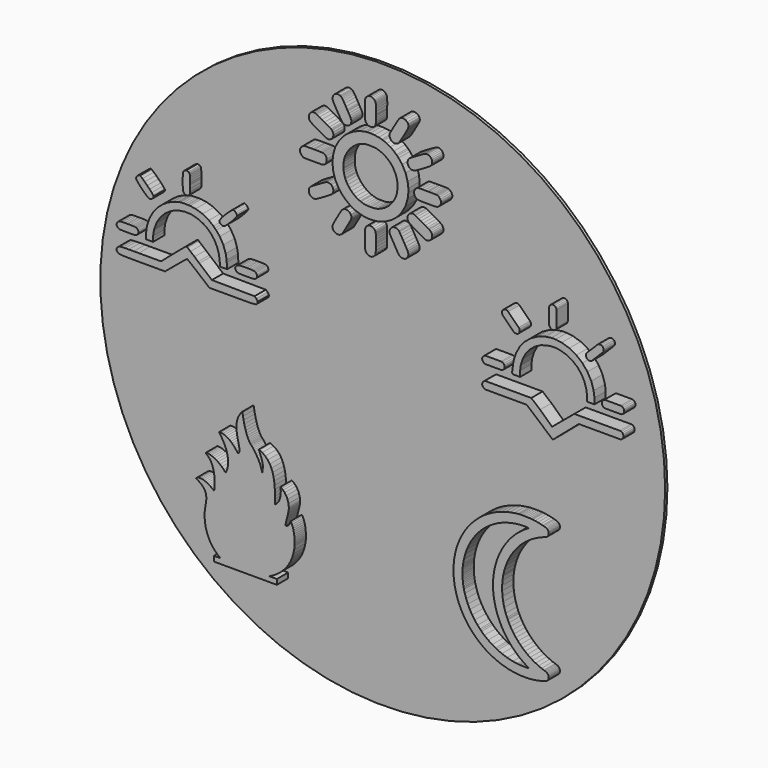
from build123d import *

# Parameters (mm, degrees)
F0_R      = 2.54
F1_DEPTH  = 0.0254
F7_DEPTH  = 0.127
F8_DEPTH  = 0.127
F9_DEPTH  = 0.127
F10_DEPTH = 0.127
F11_DEPTH = 0.127


# Not quite as in the source:
# - a feature names something its author has since deleted; it is built from what else it names


with BuildPart() as f1:
    # F0 (on Front) → F1 (new body)
    with BuildSketch(Plane.XZ):
        Circle(F0_R)
    extrude(amount=F1_DEPTH)


with BuildPart() as f7:
    # F2 (on face) → F7 (new body)
    with BuildSketch(Plane.XZ.offset(0.0254)):
        Polygon((1.2692778416, 0.5493445328), (1.270369884, 0.5471772229), (1.3371176617, 0.5471772229), (1.3371176617, 0.5513474493), (1.3371176617, 0.5638111588), (1.3371176617, 0.5764996513), (1.3371176617, 0.5807235571), (1.3371176617, 0.595958471), (1.3431767355, 0.6416296629), (1.3605789593, 0.6982145687), (1.3881735787, 0.74934765), (1.4247930644, 0.793831183), (1.4692464026, 0.8304707985), (1.520372774, 0.8581023226), (1.5770180693, 0.8755582259), (1.6227597155, 0.8816206547), (1.6380080493, 0.8816206547), (1.6532463181, 0.8816206547), (1.6989846094, 0.8755582259), (1.7556533894, 0.8581560021), (1.8067797608, 0.8305613827), (1.8512263891, 0.7939586718), (1.8878525848, 0.7495086886), (1.9154472041, 0.6983588324), (1.932846073, 0.6417168921), (1.9389252766, 0.5959786008), (1.9389252766, 0.5807235571), (1.9389252766, 0.5765768156), (1.9389252766, 0.5640862663), (1.9389252766, 0.5514179036), (1.9389252766, 0.5471772229), (2.0056723833, 0.5471772229), (2.0056723833, 0.5513474493), (2.0056723833, 0.5638111588), (2.0056723833, 0.5764996513), (2.0056723833, 0.5807235571), (2.0056723833, 0.599092012), (1.9981002185, 0.6541302771), (1.9764170543, 0.7228064909), (1.9422198561, 0.7852022029), (1.8970586195, 0.8397741274), (1.84249005, 0.8849487839), (1.7800775632, 0.9191325622), (1.7113979944, 0.9408123714), (1.6563597293, 0.9483677614), (1.6380080493, 0.9483677614), (1.6196630792, 0.9483677614), (1.5646181041, 0.9408123714), (1.4959452453, 0.9191325622), (1.4335327585, 0.8849487839), (1.378960834, 0.8397741274), (1.3338029524, 0.7852022029), (1.2996020637, 0.7228064909), (1.277923932, 0.6541302771), (1.270369884, 0.599092012), (1.270369884, 0.5807235571), (1.2692959584, 0.5785226975), (1.2666203707, 0.5716047516), (1.2653827227, 0.5638111588), (1.2666203707, 0.5561148601), align=None)
    extrude(amount=F7_DEPTH)


with BuildPart() as f7b:
    # F2 (on face) → F7, piece 2 (new body)
    with BuildSketch(Plane.XZ.offset(0.0254)):
        Polygon((1.1833466872, 0.9815651788), (1.2770137289, 0.8879179314), (1.2793071857, 0.8856063578), (1.2880441958, 0.8804564805), (1.3004213471, 0.8779570286), (1.3127803816, 0.8804564805), (1.3215173917, 0.8856063578), (1.3238474176, 0.8879179314), (1.3261589912, 0.89022615), (1.331309875, 0.898965844), (1.3337861775, 0.9113255495), (1.331309875, 0.9237020299), (1.3261589912, 0.9324215941), (1.3238474176, 0.9347331677), (1.2301803758, 1.028400545), (1.2278503499, 1.0307322484), (1.2191136753, 1.0358787707), (1.2067546408, 1.0383715126), (1.1943952708, 1.0358787707), (1.1856585962, 1.0307322484), (1.1833466872, 1.028400545), (1.1810351136, 1.0260856164), (1.175866113, 1.0173660522), (1.1733904814, 1.0049895718), (1.175866113, 0.9926332213), (1.1810169967, 0.9838968822), align=None)
    extrude(amount=F7_DEPTH)


with BuildPart() as f7c:
    # F2 (on face) → F7, piece 3 (new body)
    with BuildSketch(Plane.XZ.offset(0.0254)):
        Polygon((1.0261737742, 0.5471772229), (1.0295773901, 0.5471772229), (1.1630883783, 0.5471772229), (1.1664916588, 0.5471772229), (1.1767212945, 0.5495827356), (1.1873149444, 0.5563530629), (1.1941768623, 0.5669446998), (1.1966343771, 0.577284714), (1.1966343771, 0.5807235571), (1.1966343771, 0.5841791751), (1.1942318838, 0.5945191893), (1.1874420977, 0.6051141812), (1.1768669002, 0.6118878634), (1.166528228, 0.6142732463), (1.1630883783, 0.6142732463), (1.0295773901, 0.6142732463), (1.0261553218, 0.6142732463), (1.0159260216, 0.610958537), (1.0053327072, 0.6026214393), (0.9984704538, 0.5917177903), (0.9960313914, 0.5834712767), (0.9960313914, 0.5807235571), (0.9960860774, 0.577284714), (0.9986160595, 0.5669446998), (1.0054598606, 0.5563530629), (1.0159807076, 0.5495827356), align=None)
    extrude(amount=F7_DEPTH)


with BuildPart() as f7d:
    # F2 (on face) → F7, piece 4 (new body)
    with BuildSketch(Plane.XZ.offset(0.0254)):
        Polygon((2.2362157826, 0.4133206729), (2.232830619, 0.4133206729), (1.8249804672, 0.4133206729), (1.7445987668, 0.3465749082), (1.6243969404, 0.2462821383), (1.5174405312, 0.3465749082), (1.4374278774, 0.4133206729), (1.0295773901, 0.4133206729), (1.0268652333, 0.4133206729), (1.0187290981, 0.41093529), (1.0078261201, 0.4041649627), (0.9993987737, 0.3935733259), (0.9960313914, 0.3832333116), (0.9960313914, 0.3797743387), (0.9960313914, 0.3763348246), (0.9993440877, 0.3659964878), (1.0076805145, 0.3554025025), (1.0185834925, 0.3486315042), (1.0268289996, 0.3462290109), (1.0295773901, 0.3462290109), (1.3972387047, 0.3462290109), (1.631019649, 0.1456260253), (1.8648240781, 0.3462290109), (2.2324850572, 0.3462290109), (2.2358869957, 0.3462290109), (2.2461162959, 0.3486315042), (2.2567112877, 0.3554025025), (2.2635721992, 0.3659964878), (2.2660313914, 0.3763348246), (2.2660313914, 0.3797743387), (2.2660313914, 0.3832333116), (2.2636258787, 0.3935733259), (2.2568924561, 0.4041649627), (2.2464081782, 0.41093529), align=None)
    extrude(amount=F7_DEPTH)


with BuildPart() as f7e:
    # F2 (on face) → F7, piece 5 (new body)
    with BuildSketch(Plane.XZ.offset(0.0254)):
        Polygon((2.072416135, 0.5830888102), (2.072416135, 0.5803779953), (2.072416135, 0.5769760569), (2.0748015179, 0.5667232718), (2.081591975, 0.556131635), (2.0921634821, 0.5492707235), (2.1025034963, 0.5468148863), (2.1059624692, 0.5468148863), (2.2394768124, 0.5468148863), (2.2428787509, 0.5468148863), (2.2531046962, 0.549217044), (2.263703043, 0.5560075011), (2.2705605994, 0.5665790082), (2.2730197917, 0.5769391522), (2.2730197917, 0.5803779953), (2.2730197917, 0.5838336133), (2.2706176339, 0.5941736275), (2.2638271768, 0.6047518445), (2.2532556698, 0.6115423016), (2.2429156555, 0.6139209746), (2.2394768124, 0.6139209746), (2.1059624692, 0.6139209746), (2.1025034963, 0.6139209746), (2.0921634821, 0.6105592957), (2.081591975, 0.6021282589), (2.0748015179, 0.5912246099), align=None)
    extrude(amount=F7_DEPTH)


with BuildPart() as f7f:
    # F2 (on face) → F7, piece 6 (new body)
    with BuildSketch(Plane.XZ.offset(0.0254)):
        Polygon((1.984227422, 0.8856063578), (1.9853915962, 0.8879179314), (2.0790623284, 0.9815651788), (2.081373902, 0.9838968822), (2.0865204244, 0.9926332213), (2.0890198762, 1.0049895718), (2.0865204244, 1.0173492773), (2.081373902, 1.0260856164), (2.0790623284, 1.028400545), (2.076730625, 1.0307322484), (2.067994286, 1.0358787707), (2.0556345805, 1.0383715126), (2.043274875, 1.0358787707), (2.0345385359, 1.0307322484), (2.0322269623, 1.028400545), (1.9385763599, 0.9347331677), (1.9362647863, 0.9324215941), (1.9310981342, 0.9237020299), (1.9286053922, 0.9113255495), (1.9310981342, 0.898965844), (1.9362480114, 0.89022615), (1.9385763599, 0.8879179314), (1.9410556819, 0.8854989988), (1.9507012176, 0.8804564805), (1.9645874339, 0.8779570286), (1.9771886972, 0.8804564805), align=None)
    extrude(amount=F7_DEPTH)


with BuildPart() as f7g:
    # F2 (on face) → F7, piece 7 (new body)
    with BuildSketch(Plane.XZ.offset(0.0254)):
        Polygon((1.6286208462, 1.0147659513), (1.6313886956, 1.0147659513), (1.6347906341, 1.0147659513), (1.6450165793, 1.017164754), (1.6556149262, 1.0239552111), (1.6624724826, 1.0345334281), (1.6649316749, 1.0448902172), (1.6649316749, 1.0483290603), (1.6649316749, 1.1818199187), (1.6649316749, 1.185245342), (1.6625295171, 1.1954746422), (1.65573906, 1.2060662791), (1.6451675529, 1.2129305455), (1.6348275387, 1.2153696079), (1.6313886956, 1.2153696079), (1.6286577509, 1.2153696079), (1.6205219513, 1.212984225), (1.6096183023, 1.2062138977), (1.6011872654, 1.1956189059), (1.5978188766, 1.1852788917), (1.5978188766, 1.1818199187), (1.5978188766, 1.0483290603), (1.5978188766, 1.0449237669), (1.6011335859, 1.0346776918), (1.6094874585, 1.0240860549), (1.6203709777, 1.0172217885), align=None)
    extrude(amount=F7_DEPTH)


with BuildPart() as f8:
    # F3 (on face) → F8 (new body)
    with BuildSketch(Plane.XZ.offset(0.0254)):
        Polygon((-1.7690962786, 0.5183341948), (-1.7800488386, 0.5088888379), (-1.8924155646, 0.4123955589), (-2.0774647861, 0.4123955589), (-2.0923647631, 0.4123955589), (-2.1369972622, 0.412351013), (-2.1824724545, 0.4121291011), (-2.2159962788, 0.4116194801), (-2.2396766941, 0.4106881038), (-2.2556404589, 0.4092471066), (-2.2660171921, 0.4071403735), (-2.2728903321, 0.404258379), (-2.2770809123, 0.4014867275), (-2.2783890894, 0.4004666682), (-2.281249424, 0.3982716607), (-2.288521842, 0.389890909), (-2.2924463731, 0.3786935512), (-2.2902292971, 0.367208893), (-2.2843091932, 0.3581399282), (-2.2818035908, 0.3556347344), (-2.2808280773, 0.3546588123), (-2.2775243276, 0.3520649355), (-2.2712274229, 0.3493153525), (-2.2606071179, 0.3473201885), (-2.2434234505, 0.3459233284), (-2.2173931388, 0.3450360893), (-2.1802108326, 0.3445485369), (-2.1295916152, 0.3443486936), (-2.0798596369, 0.3442824878), (-2.0632746822, 0.3442824878), (-1.8560996549, 0.3442824878), (-1.7590264623, 0.4254548519), (-1.7495614889, 0.4333259827), (-1.721068486, 0.4568282146), (-1.6894531861, 0.4827252974), (-1.6674990249, 0.5004189945), (-1.6590067042, 0.5070485627), (-1.6585653324, 0.5071813829), (-1.6580136176, 0.5074699093), (-1.6492311358, 0.5013724393), (-1.6268560367, 0.4841221574), (-1.594799365, 0.4582696206), (-1.5659753332, 0.434545068), (-1.5563959301, 0.4265856629), (-1.4576430725, 0.3442824878), (-1.2493360083, 0.3442824878), (-1.233078813, 0.3442824878), (-1.1842581858, 0.344326625), (-1.1341052695, 0.3445264683), (-1.0968093509, 0.3449919521), (-1.0703147815, 0.3457900995), (-1.0525986071, 0.3470320707), (-1.0415561381, 0.3488498687), (-1.0351725939, 0.351311334), (-1.0321810738, 0.3535946158), (-1.0313596318, 0.3545039235), (-1.0292304214, 0.3568317511), (-1.0240402158, 0.364968931), (-1.0224463731, 0.3747914974), (-1.0265903641, 0.3848351583), (-1.0337749164, 0.3934386393), (-1.036484449, 0.3959438331), (-1.0512254504, 0.4095572929), (-1.4349369446, 0.412972203), (-1.5473314607, 0.5088888379), (-1.5582186322, 0.5183562634), (-1.5910517913, 0.5464928995), (-1.6276366109, 0.5771551631), (-1.6531789615, 0.5978219899), (-1.6610746129, 0.6053825256), (-1.6636901496, 0.6053825256), (-1.6663015995, 0.6053825256), (-1.6741277758, 0.5978219899), (-1.6995189156, 0.5771551631), (-1.7360792146, 0.5464928995), align=None)
    extrude(amount=F8_DEPTH)


with BuildPart() as f8b:
    # F3 (on face) → F8, piece 2 (new body)
    with BuildSketch(Plane.XZ.offset(0.0254)):
        Polygon((-1.2100866107, 0.600081977), (-1.2112840361, 0.5991297582), (-1.2141447793, 0.5969351594), (-1.2214233275, 0.5885531817), (-1.2253425458, 0.5773554152), (-1.2231234264, 0.5658715744), (-1.2172057746, 0.5568030182), (-1.2147005809, 0.5542978245), (-1.2137933166, 0.5533864734), (-1.2108426642, 0.5508812796), (-1.2063839915, 0.5482224231), (-1.2006420711, 0.5462264417), (-1.1928608494, 0.544807513), (-1.1823087936, 0.5438544768), (-1.168246197, 0.5432999013), (-1.1499823947, 0.5430338522), (-1.1325522946, 0.5429451691), (-1.1267204651, 0.5429451691), (-1.1209172431, 0.5429451691), (-1.1034830563, 0.5430338522), (-1.0852110803, 0.5432999013), (-1.0711566574, 0.5438544768), (-1.0606086883, 0.544807513), (-1.052819293, 0.5462264417), (-1.0470814594, 0.5482224231), (-1.0426268735, 0.5508812796), (-1.0396517005, 0.5533864734), (-1.0387444362, 0.5542978245), (-1.0371914612, 0.5558712333), (-1.0307384418, 0.5656508884), (-1.0273913722, 0.574163643), (-1.0273913722, 0.5769998657), (-1.0273913722, 0.579840175), (-1.0307384418, 0.5883529296), (-1.0371914612, 0.5981530187), (-1.0387444362, 0.5997059936), (-1.0396721343, 0.6006377786), (-1.0426268735, 0.6031429723), (-1.0470119842, 0.6058034636), (-1.0526435617, 0.6077978103), (-1.0601795768, 0.6092159216), (-1.0703352154, 0.6101722272), (-1.0837766219, 0.610723942), (-1.1012026352, 0.6109936692), (-1.1177867726, 0.6110590576), (-1.1233039203, 0.6110590576), (-1.1288047209, 0.6110590576), (-1.1452826021, 0.6109936692), (-1.1626840948, 0.610723942), (-1.1762562782, 0.6101477066), (-1.1866734704, 0.6091505332), (-1.1946835516, 0.6076670335), (-1.2009771868, 0.605558257), (-1.2062777353, 0.6027424683), align=None)
    extrude(amount=F8_DEPTH)


with BuildPart() as f8c:
    # F3 (on face) → F8, piece 3 (new body)
    with BuildSketch(Plane.XZ.offset(0.0254)):
        Polygon((-1.3050305929, 0.9794451415), (-1.3106172158, 0.9737481756), (-1.319975933, 0.9644180658), (-1.3470671718, 0.9354183026), (-1.3649876849, 0.9101211586), (-1.3665120524, 0.8932223394), (-1.3574884508, 0.8825803745), (-1.3537653978, 0.8800915279), (-1.3517914849, 0.8788328008), (-1.3401523466, 0.8745089917), (-1.3285132083, 0.8738673679), (-1.3265147748, 0.8744149959), (-1.3237194199, 0.8751097478), (-1.3160934958, 0.8803367344), (-1.3002613252, 0.8932427733), (-1.2811270395, 0.9109834684), (-1.2607503739, 0.9313356133), (-1.2412646255, 0.9521781714), (-1.2247663104, 0.9713369777), (-1.2133274241, 0.9866337806), (-1.2090240489, 0.9935976471), (-1.2090240489, 0.9959025888), (-1.2090240489, 0.9987837659), (-1.212526416, 1.0073864296), (-1.2212394226, 1.0188294027), (-1.2325066643, 1.0276077977), (-1.2408845553, 1.031089731), (-1.2436594763, 1.031089731), (-1.2457886866, 1.031089731), (-1.2521272763, 1.0266106244), (-1.2675548561, 1.0143502961), (-1.2878048316, 0.9961477954), align=None)
    extrude(amount=F8_DEPTH)


with BuildPart() as f8d:
    # F3 (on face) → F8, piece 4 (new body)
    with BuildSketch(Plane.XZ.offset(0.0254)):
        Polygon((-1.6824198445, 1.1991093565), (-1.6858159554, 1.1956928117), (-1.6867232197, 1.1947855474), (-1.6892488473, 1.1918348951), (-1.6919134253, 1.1873803091), (-1.6939077721, 1.1816343019), (-1.6953299701, 1.1738530802), (-1.696282189, 1.1633010244), (-1.6968339037, 1.1492425146), (-1.6970995442, 1.1309746255), (-1.6971690194, 1.1135445254), (-1.6971690194, 1.1077167827), (-1.6971690194, 1.1019094739), (-1.6970995442, 1.0844752871), (-1.6968339037, 1.0662114847), (-1.696282189, 1.052152975), (-1.6953299701, 1.0416009191), (-1.6939077721, 1.0338115238), (-1.6919134253, 1.0280736902), (-1.6892488473, 1.0236191043), (-1.6867477403, 1.0206684519), (-1.6858159554, 1.019736667), (-1.6831309435, 1.0170516551), (-1.6730897346, 1.0109991397), (-1.6597178033, 1.0085348137), (-1.6471877478, 1.0122415196), (-1.6388956791, 1.0191399977), (-1.6369912414, 1.0219966542), (-1.6355526962, 1.0243669843), (-1.6326020439, 1.0323770654), (-1.6302071931, 1.0483359261), (-1.629496094, 1.0739927064), (-1.6299415526, 1.1035482711), (-1.6301826724, 1.1133892279), (-1.6303420567, 1.1192210574), (-1.6308242963, 1.1366756781), (-1.6315190482, 1.1549640011), (-1.6323568373, 1.1689979902), (-1.6334643536, 1.1794683106), (-1.6349519401, 1.1870043257), (-1.6369054191, 1.1923457421), (-1.6394514806, 1.1961587042), (-1.6418258975, 1.1984636459), (-1.6426677734, 1.1991093565), (-1.6465011694, 1.2018148023), (-1.6649039221, 1.2065595493), align=None)
    extrude(amount=F8_DEPTH)


with BuildPart() as f8e:
    # F3 (on face) → F8, piece 5 (new body)
    with BuildSketch(Plane.XZ.offset(0.0254)):
        Polygon((-2.1042932451, 1.021305989), (-2.1058454027, 1.019736667), (-2.1074192202, 1.0181877788), (-2.113871831, 1.0080321402), (-2.1171972407, 0.9989390634), (-2.1171972407, 0.9959025888), (-2.1171972407, 0.9933524405), (-2.1125857225, 0.9857019957), (-2.1002575537, 0.9693834987), (-2.0825421967, 0.9492724736), (-2.0617229333, 0.927653428), (-2.0401051138, 0.9068313038), (-2.0199944973, 0.8891192163), (-2.0036760004, 0.8767894128), (-1.9960263729, 0.8721590955), (-1.9934545647, 0.8721590955), (-1.9905276156, 0.8721590955), (-1.9817475859, 0.8753059131), (-1.9703512021, 0.883172957), (-1.9617039925, 0.8934879799), (-1.9582674225, 0.9013386768), (-1.9582674225, 0.9039542135), (-1.9582674225, 0.9062591552), (-1.963167467, 0.9131780671), (-1.9761376683, 0.9293167459), (-1.9946961273, 0.9499140974), (-2.0163805612, 0.9724199734), (-2.0386857764, 0.9943087461), (-2.059084102, 1.0130588748), (-2.0751144812, 1.0261651658), (-2.0819880299, 1.031089731), (-2.0842717204, 1.031089731), (-2.0869326203, 1.031089731), (-2.0948478882, 1.0277630952), align=None)
    extrude(amount=F8_DEPTH)


with BuildPart() as f8f:
    # F3 (on face) → F8, piece 6 (new body)
    with BuildSketch(Plane.XZ.offset(0.0254)):
        Polygon((-2.2796972664, 0.5990848037), (-2.2806727799, 0.5979977212), (-2.2831563137, 0.5953617506), (-2.2894086724, 0.5863136284), (-2.2925350561, 0.5755163659), (-2.2900294537, 0.5650501324), (-2.2841759643, 0.5566681546), (-2.2818035908, 0.5542978245), (-2.2808946918, 0.5533864734), (-2.2779456742, 0.5508812796), (-2.2734890448, 0.5482224231), (-2.2677467157, 0.5462264417), (-2.259964268, 0.544807513), (-2.2494101688, 0.5438544768), (-2.235352885, 0.5432999013), (-2.2170833612, 0.5430338522), (-2.1996553045, 0.5429451691), (-2.1938242924, 0.5429451691), (-2.1880157576, 0.5429451691), (-2.1705877009, 0.5430338522), (-2.1523181771, 0.5432999013), (-2.1382608933, 0.5438544768), (-2.1277072027, 0.544807513), (-2.119924755, 0.5462264417), (-2.1141816086, 0.5482224231), (-2.1097253879, 0.5508812796), (-2.1067547104, 0.5533864734), (-2.1058454027, 0.5542978245), (-2.1034726205, 0.5566926752), (-2.0978631116, 0.565385248), (-2.0952026204, 0.5769998657), (-2.0978631116, 0.5886185701), (-2.1034726205, 0.5973315767), (-2.1058454027, 0.5997059936), (-2.106776779, 0.6006377786), (-2.1097253879, 0.6031429723), (-2.11415954, 0.6058034636), (-2.1198577319, 0.6077978103), (-2.1275739738, 0.6092159216), (-2.1379952529, 0.6101722272), (-2.1518306247, 0.610723942), (-2.1698340994, 0.6109936692), (-2.1869956982, 0.6110590576), (-2.1926938901, 0.6110590576), (-2.198702677, 0.6110590576), (-2.2167057431, 0.6110141031), (-2.235264202, 0.6107934172), (-2.2492328027, 0.6102376156), (-2.259476307, 0.6092159216), (-2.2668594767, 0.6076220789), (-2.2722916194, 0.6053171372), (-2.27659336, 0.602145799), align=None)
    extrude(amount=F8_DEPTH)


with BuildPart() as f8g:
    # F3 (on face) → F8, piece 7 (new body)
    with BuildSketch(Plane.XZ.offset(0.0254)):
        Polygon((-1.7252819521, 0.9353038729), (-1.728387902, 0.9345927738), (-1.7422665936, 0.9316257744), (-1.7830607925, 0.919075285), (-1.8327723369, 0.8967247066), (-1.8785360556, 0.8669239353), (-1.911351233, 0.8391665521), (-1.9213728253, 0.8290068267), (-1.9336343796, 0.8166851968), (-1.9655623178, 0.774865217), (-1.9985765212, 0.7138046954), (-2.0192408958, 0.6484857531), (-2.026380085, 0.5982878823), (-2.026380085, 0.5815484474), (-2.026380085, 0.5429451691), (-1.9639431371, 0.5429451691), (-1.9639431371, 0.5701953835), (-1.963899, 0.5874456654), (-1.9560724151, 0.6391270358), (-1.9340773861, 0.7022064248), (-1.8998653487, 0.7578805756), (-1.8552536922, 0.8045556453), (-1.8021296898, 0.8406745724), (-1.7423769365, 0.8646639481), (-1.6778140478, 0.8749258429), (-1.6268110821, 0.8730867936), (-1.6103168538, 0.8698991083), (-1.5976151537, 0.8674143484), (-1.5601884583, 0.8560367638), (-1.514800723, 0.8351942057), (-1.4745337181, 0.8078577604), (-1.4398369891, 0.7744687997), (-1.4111437341, 0.7355340839), (-1.388842197, 0.6914990715), (-1.3733655759, 0.6428541756), (-1.3662014574, 0.6033432244), (-1.3651184618, 0.5900612021), (-1.3611502022, 0.5429451691), (-1.2981321148, 0.5429451691), (-1.3015486596, 0.595737734), (-1.3024804446, 0.6126324664), (-1.3110422405, 0.6629856347), (-1.3319215796, 0.7245120488), (-1.364292933, 0.780852344), (-1.396288303, 0.8205390266), (-1.4082666438, 0.8324233715), (-1.4206822695, 0.8446387452), (-1.461832018, 0.8773452143), (-1.5188139371, 0.9094100596), (-1.5806754668, 0.9292554443), (-1.6318255564, 0.9368364139), (-1.6489205408, 0.9374330832), (-1.6548872339, 0.9376537691), (-1.672754619, 0.937874455), (-1.6956814329, 0.9375229923), (-1.7151058797, 0.9364113892), align=None)
    extrude(amount=F8_DEPTH)


with BuildPart() as f9:
    # F4 (on face) → F9 (new body)
    with BuildSketch(Plane.XZ.offset(0.0254)):
        Polygon((-0.4048340655, 1.5237536493), (-0.4071004206, 1.522699946), (-0.4093578459, 1.5216623162), (-0.4159175954, 1.5180654375), (-0.4318374447, 1.5091911127), (-0.452495387, 1.4974378561), (-0.4754977298, 1.4841915556), (-0.4984904286, 1.4708291692), (-0.5190706826, 1.4587312267), (-0.5348837329, 1.4492621846), (-0.5414336597, 1.4452813292), (-0.5435266002, 1.4438168603), (-0.5464139258, 1.4417648178), (-0.5539329024, 1.4339727712), (-0.5606573153, 1.4224231116), (-0.5638062808, 1.4098858284), (-0.5634960634, 1.397094942), (-0.5598434635, 1.384780901), (-0.5529443858, 1.3736759399), (-0.5429258107, 1.3644997916), (-0.5333044281, 1.3591526939), (-0.529884, 1.3579882625), (-0.5278783919, 1.3573113921), (-0.521434907, 1.3564005638), (-0.5117456588, 1.3567881123), (-0.5014554425, 1.3590848283), (-0.4936555378, 1.3619726897), (-0.4911846929, 1.3632032008), (-0.487871064, 1.3648498354), (-0.4780750167, 1.3701308534), (-0.4599659648, 1.380246405), (-0.4388240333, 1.3923943538), (-0.4166248267, 1.4054084824), (-0.395347164, 1.4181029281), (-0.3769573627, 1.4293025439), (-0.36343067, 1.4378571859), (-0.3582371629, 1.4412004614), (-0.3567459049, 1.4425774194), (-0.3528597043, 1.4462118028), (-0.3446443905, 1.4608118442), (-0.341960126, 1.4816448084), (-0.3483448536, 1.5017383943), (-0.3589836849, 1.5147810979), (-0.3634413856, 1.5177386109), (-0.3657648907, 1.5192691596), (-0.3736158731, 1.5224963491), (-0.3854637844, 1.525053812), (-0.3972170409, 1.5252074027), align=None)
    extrude(amount=F9_DEPTH)


with BuildPart() as f9b:
    # F4 (on face) → F9, piece 2 (new body)
    with BuildSketch(Plane.XZ.offset(0.0254)):
        Polygon((-0.6034937473, 1.7449509729), (-0.6047923027, 1.7447009417), (-0.6085225909, 1.7439347743), (-0.6190451577, 1.7383840797), (-0.6315251123, 1.7268719248), (-0.6403713979, 1.7124344038), (-0.6437336044, 1.7010972708), (-0.6437336044, 1.6973200124), (-0.6436852055, 1.6937552806), (-0.640652326, 1.683066443), (-0.6328524213, 1.6690164705), (-0.6219326619, 1.6575257468), (-0.6128150924, 1.6518178896), (-0.6095011062, 1.6509374223), (-0.6085709899, 1.6506266691), (-0.6003253151, 1.6501033894), (-0.5803265625, 1.649483669), (-0.5524696836, 1.6490961205), (-0.5279073241, 1.6489496736), (-0.5197102269, 1.6489496736), (-0.5129565246, 1.6489496736), (-0.4926866666, 1.6489693189), (-0.4721064126, 1.6490461142), (-0.4569423721, 1.6492604267), (-0.4461678095, 1.6496676206), (-0.4387365224, 1.6503462769), (-0.4336305263, 1.6513642614), (-0.429792546, 1.6527769382), (-0.4270797065, 1.6541646119), (-0.4261992392, 1.6546575307), (-0.4216450978, 1.6570506873), (-0.4102686742, 1.6686467813), (-0.4019854948, 1.6878706156), (-0.4020337151, 1.708898247), (-0.4078469426, 1.7242376666), (-0.4110634165, 1.7283256782), (-0.4116831369, 1.7291097048), (-0.4138155466, 1.7312313989), (-0.4176142363, 1.7344693041), (-0.4219254901, 1.7376071968), (-0.4251026734, 1.7396431659), (-0.4261992392, 1.7402343113), (-0.4270904221, 1.7406879395), (-0.4298229069, 1.7419684569), (-0.4337073216, 1.7432954086), (-0.438804388, 1.7442741025), (-0.4460713688, 1.7449813339), (-0.4564673126, 1.7454546074), (-0.4709532326, 1.7457850059), (-0.490477283, 1.7459993184), (-0.5096139635, 1.7461439794), (-0.5159894041, 1.7461814841), (-0.5238862852, 1.7462314903), (-0.5475574617, 1.7462011294), (-0.574813194, 1.7459118075), (-0.5948607027, 1.7453885277), align=None)
    extrude(amount=F9_DEPTH)


with BuildPart() as f9c:
    # F4 (on face) → F9, piece 3 (new body)
    with BuildSketch(Plane.XZ.offset(0.0254)):
        Polygon((-0.5287988643, 2.0373857827), (-0.530872338, 2.0366499763), (-0.5360076235, 2.0348568948), (-0.5497664882, 2.0248181385), (-0.5611029068, 2.0068837514), (-0.5638353916, 1.9857900403), (-0.5596980882, 1.9691736752), (-0.5569172044, 1.9644641572), (-0.5563648139, 1.9635140383), (-0.5544463595, 1.9607922692), (-0.5509777112, 1.9570525155), (-0.5457358052, 1.9527412617), (-0.5379746554, 1.9473530874), (-0.5269288088, 1.9403861441), (-0.5118229899, 1.9313260818), (-0.4918921029, 1.9196799815), (-0.472765245, 1.908616097), (-0.4663799817, 1.9049317073), (-0.4617001103, 1.9022581585), (-0.4476126331, 1.8942553713), (-0.4325732511, 1.8858453903), (-0.4207146243, 1.8794499471), (-0.4114706103, 1.8747993651), (-0.4042911404, 1.8716400412), (-0.3986136442, 1.8697112284), (-0.3938666216, 1.8687414642), (-0.3905787102, 1.8684717876), (-0.3894857162, 1.8684717876), (-0.3872390065, 1.8684717876), (-0.3804631586, 1.8697987393), (-0.3704851242, 1.8732491711), (-0.3612036056, 1.87810335), (-0.3557564954, 1.88200741), (-0.3542652373, 1.8836076102), (-0.3510576931, 1.8870848311), (-0.3443443529, 1.9002132597), (-0.3416493728, 1.9189816798), (-0.3460767126, 1.9374304171), (-0.3539759154, 1.9498998347), (-0.3574924269, 1.9530609445), (-0.3591301318, 1.9545414869), (-0.3647969124, 1.95812765), (-0.3794362444, 1.967227003), (-0.3991851443, 1.9790659845), (-0.4217986885, 1.99234086), (-0.4450444546, 2.0057514668), (-0.4666707324, 2.0179762109), (-0.4844508145, 2.0277256453), (-0.4931711915, 2.0323083616), (-0.4961456709, 2.0336763899), (-0.4984323856, 2.0347408088), (-0.5055541697, 2.0373572077), (-0.5140711284, 2.039071708), (-0.5223069804, 2.0388395361), align=None)
    extrude(amount=F9_DEPTH)


with BuildPart() as f9d:
    # F4 (on face) → F9, piece 4 (new body)
    with BuildSketch(Plane.XZ.offset(0.0254)):
        Polygon((-0.3197894944, 2.249406958), (-0.3232595715, 2.2477299624), (-0.32749403, 2.245618984), (-0.3385186239, 2.2359409872), (-0.3474804597, 2.2199246972), (-0.34959501, 2.2014545286), (-0.3464642611, 2.1866687498), (-0.3443443529, 2.1822503397), (-0.3425602011, 2.178626672), (-0.3368059096, 2.1679378343), (-0.325972411, 2.1486675657), (-0.3130743684, 2.1264701451), (-0.2993262193, 2.1033422508), (-0.2859459735, 2.0813287818), (-0.274164142, 2.0624317741), (-0.2651915906, 2.0486925548), (-0.2617411588, 2.0434811883), (-0.2602481148, 2.0421042303), (-0.2572263081, 2.0394771158), (-0.2463445892, 2.0336656743), (-0.2308319336, 2.0303313285), (-0.2150853202, 2.0322029913), (-0.2037213982, 2.0370268092), (-0.2004763492, 2.0393717455), (-0.1972598753, 2.0417381131), (-0.1859709626, 2.05640602), (-0.1811257134, 2.0737796228), (-0.1811257134, 2.0795642752), (-0.1811257134, 2.0807162051), (-0.1812632306, 2.0841559213), (-0.1818633057, 2.0885368266), (-0.1832759825, 2.0934481555), (-0.185844161, 2.0996221424), (-0.1899053835, 2.10778745), (-0.195775761, 2.1186691688), (-0.2038267685, 2.1330013195), (-0.2117259713, 2.1468851998), (-0.2143602295, 2.1514982771), (-0.2182267848, 2.1582401922), (-0.2298728851, 2.178423075), (-0.2421779964, 2.1994596361), (-0.2518292041, 2.2154277058), (-0.2593872928, 2.2271220264), (-0.2654130469, 2.2353677011), (-0.270461893, 2.240968402), (-0.2750838999, 2.2447456604), (-0.2786307724, 2.2468798561), (-0.2798505679, 2.2474888608), (-0.2833295747, 2.2492337221), (-0.3015550697, 2.2527305882), align=None)
    extrude(amount=F9_DEPTH)


with BuildPart() as f9e:
    # F4 (on face) → F9, piece 5 (new body)
    with BuildSketch(Plane.XZ.offset(0.0254)):
        Polygon((-0.0360486298, 2.038123375), (-0.0446997124, 2.0371428952), (-0.0592729647, 2.0354873308), (-0.1024587261, 2.0259325637), (-0.1554885766, 2.0058675528), (-0.2042839686, 1.9766246076), (-0.2388936568, 1.9484175063), (-0.2493396068, 1.9379251218), (-0.2614518369, 1.9258628981), (-0.293423695, 1.8853024652), (-0.3246258139, 1.8279506453), (-0.3431799215, 1.7654356793), (-0.3493039022, 1.714352501), (-0.3493039022, 1.6973200124), (-0.3493039022, 1.6802964535), (-0.3431799215, 1.6292132752), (-0.3246258139, 1.5666983092), (-0.293423695, 1.5093464893), (-0.2614518369, 1.4687860564), (-0.2493396068, 1.456713117), (-0.2372755972, 1.4446116026), (-0.1967151643, 1.4126361726), (-0.1393651303, 1.3814358396), (-0.0768501643, 1.362881732), (-0.025766986, 1.3567488217), (-0.0087327114, 1.3567488217), (0.0082908475, 1.3567488217), (0.0593722398, 1.362881732), (0.1218872058, 1.3814358396), (0.1792390257, 1.4126361726), (0.2198101743, 1.4446116026), (0.231872398, 1.456713117), (0.2439739124, 1.4687771267), (0.2759493424, 1.5093464893), (0.3071496754, 1.5666983092), (0.325703783, 1.6292132752), (0.3318366933, 1.6802964535), (0.3318366933, 1.6973200124), (0.3318366933, 1.714352501), (0.325703783, 1.7654356793), (0.3071496754, 1.8279506453), (0.2759493424, 1.8853024652), (0.2439739124, 1.9258628981), (0.231872398, 1.9379251218), (0.2245875578, 1.9452599683), (0.2013025011, 1.9658393293), (0.1700432321, 1.9884064391), (0.1366444097, 2.0065051326), (0.1090695304, 2.0178994156), (0.0996612102, 2.0210212348), (0.0910958526, 2.0238787353), (0.0647496985, 2.0304188394), (0.027477177, 2.0364356638), (-0.0098007022, 2.0387806001), align=None)
        Polygon((0.0488102038, 1.9348247339), (0.0507979525, 1.9342032275), (0.0604598759, 1.9312867911), (0.0888277116, 1.9204550785), (0.121424648, 1.903392229), (0.1502103931, 1.8819609756), (0.1706165181, 1.862203146), (0.1768083644, 1.855082612), (0.1811196182, 1.8502177175), (0.1928550154, 1.8345211104), (0.2066299535, 1.8114878708), (0.2184528616, 1.7853953199), (0.2263984987, 1.763147893), (0.2286452085, 1.7556094496), (0.2293042195, 1.7533430946), (0.2308061932, 1.7463654357), (0.2321813653, 1.7350300886), (0.2328993123, 1.7194102768), (0.2331118388, 1.7028439179), (0.2331118388, 1.6973200124), (0.2331118388, 1.6903048488), (0.232735006, 1.6692397127), (0.2308454838, 1.6494158033), (0.2263109878, 1.6312188833), (0.2201566462, 1.6137863446), (0.2179760162, 1.6080231234), (0.215856108, 1.6023634866), (0.2081140678, 1.5858721372), (0.1954892736, 1.5644783885), (0.1804516775, 1.5441597744), (0.1633102467, 1.5252770542), (0.1444257406, 1.5081338375), (0.1241071265, 1.4930980273), (0.1027133778, 1.4804714472), (0.0862220284, 1.472729407), (0.0805641775, 1.4706094988), (0.0747991704, 1.4684288688), (0.0573666317, 1.4622745272), (0.0391714976, 1.4577400312), (0.0193458023, 1.455850509), (-0.0017193338, 1.4554736762), (-0.0087327114, 1.4554736762), (-0.0157585907, 1.4554736762), (-0.0368130111, 1.455850509), (-0.0566369205, 1.4577400312), (-0.0748338405, 1.4622745272), (-0.0922753089, 1.4684288688), (-0.0980296004, 1.4706094988), (-0.1036981669, 1.472729407), (-0.1201913023, 1.4804714472), (-0.1415850509, 1.4930980273), (-0.1619018791, 1.5081338375), (-0.1807863852, 1.5252770542), (-0.1979260301, 1.5441597744), (-0.2129654121, 1.5644783885), (-0.2255902063, 1.5858721372), (-0.2333322465, 1.6023634866), (-0.235443225, 1.6080231234), (-0.2373738237, 1.6131576945), (-0.2427405668, 1.6286899954), (-0.2472661331, 1.6457331996), (-0.2497860913, 1.6631353773), (-0.2508790852, 1.6794713502), (-0.2510737524, 1.6849166745), (-0.2513255697, 1.6914853537), (-0.2513523587, 1.7112056786), (-0.2497450147, 1.733353093), (-0.2459588266, 1.7539128087), (-0.2414404041, 1.7701434113), (-0.2396705397, 1.7754547902), (-0.2358021985, 1.786741917), (-0.2197466178, 1.8190656048), (-0.1919217073, 1.8578990359), (-0.1572120065, 1.8907388598), (-0.1273118362, 1.9110074676), (-0.1166337142, 1.9163474216), (-0.1131654231, 1.9180512062), (-0.1024015761, 1.9224410413), (-0.0846404249, 1.9288168392), (-0.0666846064, 1.9343496744), (-0.0556296516, 1.9372375358), (-0.0518881119, 1.9379251218), (-0.0495735366, 1.9383412453), (-0.0425101527, 1.9389716814), (-0.0298174929, 1.9395146065), (-0.0149834937, 1.9395824721), (0.0008488447, 1.9392324283), (0.0164972316, 1.9384769766), (0.030807951, 1.9373714811), (0.0426290731, 1.9359373731), align=None, mode=Mode.SUBTRACT)
    extrude(amount=F9_DEPTH)


with BuildPart() as f9f:
    # F4 (on face) → F9, piece 6 (new body)
    with BuildSketch(Plane.XZ.offset(0.0254)):
        Polygon((0.3553324908, 1.5228231757), (0.3521749528, 1.5214587193), (0.3493353117, 1.5201782019), (0.3414789714, 1.5148686089), (0.3332511561, 1.506226456), (0.3275629442, 1.4960805434), (0.3245125625, 1.4849684386), (0.324153589, 1.473416993), (0.3265663909, 1.4619852053), (0.3318277636, 1.4511892114), (0.3377088568, 1.4436918446), (0.3400252181, 1.4415772943), (0.3416522074, 1.4401074675), (0.3473207739, 1.4365195185), (0.3619601059, 1.4274219515), (0.3817072199, 1.4155829699), (0.40432255, 1.4023063085), (0.4275683161, 1.3888974876), (0.4491942367, 1.3766691717), (0.4669732473, 1.3669233092), (0.4756939814, 1.3623388069), (0.4786782835, 1.3609618489), (0.4809553541, 1.359868855), (0.4880669584, 1.3570774342), (0.4960983206, 1.3553647199), (0.5038600062, 1.3556343965), (0.5103251009, 1.3570774342), (0.51241822, 1.3577471609), (0.5164562253, 1.3590955439), (0.5277540677, 1.3657035137), (0.5388590288, 1.377435339), (0.5451580314, 1.3921050319), (0.5465814238, 1.404729826), (0.5461456549, 1.4088374829), (0.5458081127, 1.4120253819), (0.543588192, 1.4214533474), (0.5383268193, 1.4317921412), (0.5295382195, 1.4410075801), (0.5197905711, 1.4481477594), (0.51637943, 1.4502587378), (0.5128057685, 1.4524500835), (0.5020097746, 1.4588848173), (0.484259339, 1.4692789752), (0.4646086656, 1.4806375395), (0.4445418688, 1.4920907584), (0.4255216314, 1.5028153148), (0.4090517132, 1.5119718178), (0.3965894394, 1.5187155188), (0.3914155776, 1.521439074), (0.3896349977, 1.5221927397), (0.3865917597, 1.5234339665), (0.3710880338, 1.5257396121), align=None)
    extrude(amount=F9_DEPTH)


with BuildPart() as f9g:
    # F4 (on face) → F9, piece 7 (new body)
    with BuildSketch(Plane.XZ.offset(0.0254)):
        Polygon((0.2722363778, 2.2516375943), (0.2673446942, 2.25021063), (0.2663552847, 2.2499409534), (0.2635281452, 2.248690797), (0.2591865304, 2.2462190591), (0.2548842063, 2.2431383164), (0.2520659965, 2.2406987254), (0.2512212479, 2.2397950409), (0.2495656836, 2.2381484063), (0.2456884127, 2.2320833616), (0.2356800174, 2.2162313778), (0.22268732, 2.1948001245), (0.2082105084, 2.1703417066), (0.1937444124, 2.1454207308), (0.1807892197, 2.1225928741), (0.1708397604, 2.1044155994), (0.1665570816, 2.0962681513), (0.1653926501, 2.0934481555), (0.1645996938, 2.0915872084), (0.1631155795, 2.0856293199), (0.1626315903, 2.0771407577), (0.1639585421, 2.0681985672), (0.1661498878, 2.061201263), (0.1671267957, 2.0589741986), (0.1682608662, 2.0562810044), (0.1730007451, 2.0487514907), (0.1808285104, 2.0406415473), (0.1901511056, 2.0347604542), (0.2004898994, 2.0311957224), (0.2113876917, 2.0300509362), (0.2223765669, 2.0314153927), (0.2329957529, 2.0354087496), (0.2405734869, 2.0401664878), (0.242780906, 2.0421042303), (0.2440221327, 2.0432275852), (0.2487709413, 2.0496926799), (0.2587507616, 2.0648052854), (0.2718398996, 2.0860561591), (0.2833984889, 2.1055300246), (0.2871882489, 2.1120504834), (0.2912494714, 2.1191049377), (0.3034188514, 2.14027723), (0.3155971611, 2.1618942209), (0.324212525, 2.1780730312), (0.3297542899, 2.1900030956), (0.3326975153, 2.1988399157), (0.3335315483, 2.2057479231), (0.3327582372, 2.2119094084), (0.3313616339, 2.2168510982), (0.3308383541, 2.2184709438), (0.3292506554, 2.2231483149), (0.3210156963, 2.2359874215), (0.3062459909, 2.2475567265), (0.2878954802, 2.252507346), align=None)
    extrude(amount=F9_DEPTH)


with BuildPart() as f9h:
    # F4 (on face) → F9, piece 8 (new body)
    with BuildSketch(Plane.XZ.offset(0.0254)):
        Polygon((-0.0259795126, 2.3282311078), (-0.0273368253, 2.3276113874), (-0.0296603303, 2.3265541123), (-0.0361147095, 2.3221946381), (-0.0444871858, 2.3146169041), (-0.0512416025, 2.3061587028), (-0.0545348717, 2.3002097441), (-0.0551153015, 2.2980862641), (-0.0554260547, 2.2971557905), (-0.0559582641, 2.2889119017), (-0.0565797705, 2.2689129704), (-0.056965533, 2.241055913), (-0.0571030502, 2.2164939107), (-0.0571030502, 2.2082964563), (-0.0571030502, 2.2015420396), (-0.0570923346, 2.1812716458), (-0.0570155393, 2.1606922848), (-0.0568030127, 2.1455278871), (-0.0563958189, 2.1347551104), (-0.0557153766, 2.1273202514), (-0.054699178, 2.1222160413), (-0.0532847153, 2.118378061), (-0.0518988276, 2.1156759371), (-0.0513951931, 2.1147847542), (-0.0490109662, 2.1102306128), (-0.0374130862, 2.0988559751), (-0.018189252, 2.0905710098), (0.0028455232, 2.0906192301), (0.0181742271, 2.0964324576), (0.0222729543, 2.0996489315), (0.0230480513, 2.1002686519), (0.0251697454, 2.1024028475), (0.0284058647, 2.1061997513), (0.0315437574, 2.1105110051), (0.0335815124, 2.1136881884), (0.0341815875, 2.1147847542), (0.0346352156, 2.1156652215), (0.0359050174, 2.1183584157), (0.0372319692, 2.1221767506), (0.0382320943, 2.1270898655), (0.0389482554, 2.1339210775), (0.0394626055, 2.1435044196), (0.0398287227, 2.1566792826), (0.0401091149, 2.1742761275), (0.0403127118, 2.191426488), (0.0403823634, 2.1971343452), (0.0404591587, 2.2046424276), (0.04065204, 2.2271595311), (0.0406716853, 2.2507160504), (0.0403430728, 2.2687772392), (0.0395679758, 2.2823128616), (0.0382588834, 2.2923016116), (0.0363211409, 2.299723969), (0.0336672374, 2.3055479121), (0.0311383495, 2.3095019783), (0.0302078759, 2.3107414192), (0.0284433694, 2.3130756398), (0.0220300668, 2.3192389111), (0.0120413168, 2.3260879825), (0.0013917698, 2.3306617691), (-0.0062038235, 2.3323191194), (-0.0087327114, 2.3323191194), (-0.0109901368, 2.3323191194), (-0.0177641988, 2.330895727), align=None)
    extrude(amount=F9_DEPTH)


with BuildPart() as f9i:
    # F4 (on face) → F9, piece 9 (new body)
    with BuildSketch(Plane.XZ.offset(0.0254)):
        Polygon((0.4932015295, 2.038123375), (0.4898403946, 2.0373964983), (0.4888706304, 2.0372000452), (0.4859738393, 2.0365142451), (0.481992984, 2.0352337277), (0.4769923582, 2.0330923883), (0.4700843509, 2.0296151674), (0.4603759931, 2.0243341494), (0.4469653863, 2.0167867764), (0.4289720632, 2.0064979888), (0.4113662886, 1.9963717216), (0.4055048408, 1.9929891555), (0.3996630383, 1.9896476659), (0.382250145, 1.9794160283), (0.3619708215, 1.9671377061), (0.3469046504, 1.957554364), (0.3403252556, 1.9530609445), (0.3392786961, 1.9520608194), (0.3353157001, 1.9483603563), (0.3270200191, 1.9333995555), (0.3246090031, 1.9121022475), (0.3316330964, 1.8916871927), (0.3430095201, 1.8785676938), (0.3477083224, 1.8756601871), (0.3489674085, 1.8748868761), (0.3529679091, 1.8728526929), (0.3584060897, 1.8710185348), (0.364626511, 1.8700219815), (0.3703522275, 1.8697112284), (0.3722721106, 1.8697112284), (0.3735115514, 1.8697112284), (0.3772602348, 1.8697987393), (0.3818143761, 1.8703023738), (0.3867382066, 1.8716025365), (0.3928496857, 1.8740528431), (0.4009614151, 1.8780444141), (0.4118895683, 1.8839451525), (0.4264431753, 1.8921229616), (0.4406985307, 1.9002436206), (0.4454455533, 1.9029457445), (0.452226759, 1.9068319451), (0.4725739481, 1.9185369813), (0.4937176655, 1.9308795973), (0.5097035946, 1.9405522363), (0.5213693401, 1.9481263984), (0.5295685805, 1.9541842994), (0.5351192751, 1.9592885096), (0.5388804601, 1.9640194587), (0.5410503745, 1.9676699156), (0.5416772386, 1.9689307876), (0.5432274326, 1.9720704662), (0.5460688596, 1.9824003304), (0.5463778269, 1.9957520012), (0.5430845576, 2.0083482204), (0.5366891144, 2.0195371205), (0.5276683427, 2.0286846938), (0.5165258769, 2.035137287), (0.5037546358, 2.0382573203), align=None)
    extrude(amount=F9_DEPTH)


with BuildPart() as f9j:
    # F4 (on face) → F9, piece 10 (new body)
    with BuildSketch(Plane.XZ.offset(0.0254)):
        Polygon((0.4226748466, 1.7449509729), (0.4216282871, 1.7447009417), (0.4177813771, 1.7437418931), (0.4067657129, 1.7387412673), (0.3952053376, 1.7293811674), (0.3873668567, 1.7171439217), (0.3840235812, 1.7062443435), (0.3836735374, 1.7025331648), (0.3833270654, 1.6987719798), (0.3841682421, 1.6873009014), (0.3885687928, 1.6740938916), (0.3967841066, 1.6630764414), (0.4055155564, 1.6561487888), (0.4087320304, 1.6544039275), (0.409601782, 1.6539502994), (0.4122967622, 1.6526804976), (0.4161133112, 1.6513535458), (0.421028212, 1.6503534207), (0.427859424, 1.6496372596), (0.4374409801, 1.6491229095), (0.450619415, 1.6487567923), (0.468214474, 1.6484764001), (0.4853630486, 1.6482728032), (0.4910816213, 1.6482031516), (0.4985789881, 1.6481263563), (0.5210996635, 1.647933475), (0.5446543969, 1.6479138297), (0.5627137997, 1.6482424422), (0.5762512081, 1.6490175392), (0.5862399581, 1.6503266316), (0.5936605296, 1.6522643741), (0.5994844727, 1.6549182776), (0.6034385389, 1.6574489515), (0.6046886953, 1.6583776391), (0.6069854113, 1.6601510753), (0.613080817, 1.6665465185), (0.619938818, 1.6764584732), (0.6245626109, 1.6868740623), (0.6262663956, 1.6941517588), (0.6262663956, 1.6965734904), (0.6262663956, 1.699798894), (0.6241054109, 1.7094518877), (0.6181385928, 1.7220070303), (0.6090963898, 1.7330619851), (0.6008114244, 1.7398074721), (0.5977413974, 1.7414737521), (0.5970806004, 1.741850585), (0.5949696219, 1.7427346242), (0.591094137, 1.7437115321), (0.5854845064, 1.7444776994), (0.5775210098, 1.7450384839), (0.566582141, 1.745465323), (0.5520356777, 1.7457653606), (0.5332779732, 1.7459993184), (0.515575758, 1.7461439794), (0.5096839492, 1.7461814841), (0.5017097371, 1.7462314903), (0.4777888865, 1.7462011294), (0.4505801244, 1.7459118075), (0.4309205213, 1.7453885277), align=None)
    extrude(amount=F9_DEPTH)


with BuildPart() as f9k:
    # F4 (on face) → F9, piece 11 (new body)
    with BuildSketch(Plane.XZ.offset(0.0254)):
        Polygon((-0.0246436311, 1.3034475086), (-0.028578052, 1.3016847881), (-0.0305247242, 1.3008025348), (-0.0361343548, 1.2976735718), (-0.0421029588, 1.2930408492), (-0.0471410893, 1.2871401108), (-0.0508147633, 1.2813661739), (-0.0518881119, 1.2793605658), (-0.0523345964, 1.2785265329), (-0.0535454622, 1.2759297793), (-0.054815264, 1.272150735), (-0.0557653829, 1.2672394061), (-0.0564529689, 1.2603885488), (-0.0569458877, 1.2507855614), (-0.0573066472, 1.2376476673), (-0.0575870394, 1.2201486917), (-0.0577888504, 1.2031729959), (-0.0578495722, 1.197504608), (-0.0579352973, 1.1900052767), (-0.0581299645, 1.1674871016), (-0.0581496098, 1.1439321897), (-0.0578192113, 1.1258715367), (-0.0570459002, 1.1123355571), (-0.0557368078, 1.1023457355), (-0.0537990654, 1.0949235567), (-0.0511451618, 1.0891005066), (-0.048614488, 1.0851471547), (-0.0476750847, 1.0838971768), (-0.0459212938, 1.0815718859), (-0.0395062053, 1.0753996849), (-0.0295174553, 1.0685590074), (-0.0188679083, 1.0639857565), (-0.011270529, 1.0623191194), (-0.0087327114, 1.0623191194), (-0.0051661937, 1.0623675183), (0.005519072, 1.0654100419), (0.0195690445, 1.0732099466), (0.0310615542, 1.0841298845), (0.0367676254, 1.0932476327), (0.0376480927, 1.0965516176), (0.0379588459, 1.097481734), (0.0384821256, 1.1057370528), (0.039101846, 1.1257358054), (0.0394893945, 1.1535830402), (0.0396358414, 1.1781550438), (0.0396358414, 1.1863424969), (0.0396358414, 1.1931058433), (0.0396161961, 1.2133757013), (0.0395394008, 1.2339559553), (0.0393250883, 1.2491192814), (0.0389196804, 1.259893844), (0.038241024, 1.2673251311), (0.0372230395, 1.2724329132), (0.0358085768, 1.2762691075), (0.0344209031, 1.2789730173), (0.0339279843, 1.2798534846), (0.0318848715, 1.2837111103), (0.0224854809, 1.2935266243), (0.0065763472, 1.3023045085), (-0.0112812447, 1.3053173855), align=None)
    extrude(amount=F9_DEPTH)


with BuildPart() as f9l:
    # F4 (on face) → F9, piece 12 (new body)
    with BuildSketch(Plane.XZ.offset(0.0254)):
        Polygon((0.1986753866, 1.3631924852), (0.1951588751, 1.3622030756), (0.1941408906, 1.361876249), (0.1912440995, 1.3604492847), (0.1865935175, 1.3576221452), (0.1817589839, 1.3540449119), (0.1783585584, 1.3511106161), (0.1773012833, 1.3500533409), (0.1747634657, 1.3475226671), (0.1685430444, 1.3385519016), (0.1635924249, 1.3257520856), (0.162642306, 1.3123825554), (0.1645889781, 1.3022955788), (0.1658873549, 1.2992041205), (0.1667892535, 1.2970431358), (0.1701700337, 1.2908227145), (0.1787657522, 1.2752332636), (0.1903136259, 1.2548074932), (0.2034634858, 1.2318921256), (0.2168437316, 1.2088508493), (0.2290916929, 1.1880382448), (0.2388500569, 1.1718181793), (0.243180956, 1.1647839062), (0.2447686547, 1.1625261237), (0.2471225207, 1.1592028506), (0.25638618, 1.1507634017), (0.2700593196, 1.1440582769), (0.2846397156, 1.1420524901), (0.2990290163, 1.1443974265), (0.3120806496, 1.1507244682), (0.32268912, 1.1606853576), (0.3297239289, 1.1739209425), (0.3321581621, 1.1860421022), (0.3320777949, 1.1900633197), (0.3320117152, 1.1919914181), (0.3303061447, 1.2022232342), (0.3269932301, 1.21196106), (0.3261306221, 1.2136276971), (0.3244732719, 1.2169413261), (0.3191922539, 1.2267082626), (0.3090463413, 1.2448669636), (0.2968769613, 1.2661142653), (0.2838646187, 1.2884492032), (0.2711826745, 1.3098625971), (0.2600294931, 1.3283595547), (0.2515695058, 1.3419255381), (0.2483244568, 1.3470690389), (0.2470082207, 1.3485602969), (0.2447115047, 1.3511195458), (0.2363193831, 1.3574381936), (0.2236838733, 1.3627352851), (0.2097410571, 1.36437299), align=None)
    extrude(amount=F9_DEPTH)


with BuildPart() as f9m:
    # F4 (on face) → F9, piece 13 (new body)
    with BuildSketch(Plane.XZ.offset(0.0254)):
        Polygon((-0.2438157013, 1.362222721), (-0.2480983801, 1.3602278285), (-0.249221735, 1.3597224081), (-0.2524792855, 1.3579221828), (-0.2570334268, 1.3549575261), (-0.261217879, 1.3517196209), (-0.2637378372, 1.3494139752), (-0.2644754295, 1.3485602969), (-0.2659559719, 1.3469333076), (-0.269542135, 1.3412647411), (-0.2786379161, 1.3266254091), (-0.2904804695, 1.3068782951), (-0.3037535591, 1.284262965), (-0.3171641659, 1.2610189848), (-0.3293906959, 1.2393916355), (-0.3391401303, 1.2216119105), (-0.3437228466, 1.212891355), (-0.3450908749, 1.2099070529), (-0.3461945845, 1.2076299823), (-0.3489842193, 1.2005180208), (-0.3506987196, 1.1924857657), (-0.350427257, 1.1847246159), (-0.3489752896, 1.1782616642), (-0.3483055629, 1.1761687238), (-0.3469571799, 1.1721282181), (-0.3403599258, 1.1608303757), (-0.3286263145, 1.1497266648), (-0.3139584076, 1.1434285552), (-0.3013318275, 1.1420042698), (-0.2972152409, 1.1424402172), (-0.2940362716, 1.1427793668), (-0.2846083061, 1.1449980373), (-0.2742695123, 1.15025941), (-0.2650558593, 1.1590478312), (-0.2579049644, 1.168795301), (-0.255793986, 1.1722059064), (-0.253613356, 1.1757811753), (-0.2471786221, 1.1865752046), (-0.2367808924, 1.2043259974), (-0.225424114, 1.2239759564), (-0.213972681, 1.2440418603), (-0.2032463387, 1.2630620976), (-0.1940916217, 1.2795338018), (-0.1873479206, 1.2919960756), (-0.1846243655, 1.2971699374), (-0.1838599841, 1.2989523033), (-0.1829473699, 1.3011811536), (-0.1809792665, 1.3081856016), (-0.1801380898, 1.317129578), (-0.1813489556, 1.326169995), (-0.183606381, 1.3333780399), (-0.1845940045, 1.3356640402), (-0.186503172, 1.3400449456), (-0.1956793203, 1.3516803302), (-0.2112419821, 1.3616226459), (-0.229358535, 1.3647337495), align=None)
    extrude(amount=F9_DEPTH)


with BuildPart() as f10:
    # F5 (on face) → F10 (new body)
    with BuildSketch(Plane.XZ.offset(0.0254)):
        Polygon((1.3290052851, -0.5420529805), (1.3264628547, -0.5422629409), (1.3159781925, -0.5431886757), (1.284631095, -0.5471683809), (1.2439092626, -0.554440648), (1.2042525025, -0.5640892857), (1.1656102331, -0.5761429252), (1.1279375993, -0.59061111), (1.0911859285, -0.6075224712), (1.0553141829, -0.6268770087), (1.0288563011, -0.6429867026), (1.0202708268, -0.6487033535), (1.0094187338, -0.6559469895), (0.9780821343, -0.67951028), (0.9386429695, -0.7136861176), (0.902155658, -0.750992275), (0.8688101186, -0.7911615295), (0.8388210835, -0.8339171153), (0.8123784715, -0.8790204408), (0.7896846083, -0.9261861508), (0.7751038083, -0.9627555377), (0.7709399105, -0.9751785167), (0.7664572545, -0.9885835381), (0.7553455741, -1.0295907258), (0.7446433165, -1.0846986676), (0.738828366, -1.1402351195), (0.7379016768, -1.1959366767), (0.7418575229, -1.251541843), (0.7506959041, -1.3067786241), (0.7644120487, -1.3613874326), (0.7777865304, -1.4019031219), (0.7830050024, -1.4151124983), (0.7839775011, -1.4176024386), (0.787105912, -1.4250073624), (0.7921907727, -1.4363719498), (0.7980095407, -1.4487204883), (0.8043112178, -1.4615509815), (0.8108514863, -1.4743767029), (0.8173755306, -1.4867051997), (0.8236399874, -1.4980440192), (0.8279174547, -1.5054537149), (0.829397676, -1.5078978456), (0.833990084, -1.5155089125), (0.8486014237, -1.5378515692), (0.8692414919, -1.5664634545), (0.8912921126, -1.5937344559), (0.9147427879, -1.6196540754), (0.9395753848, -1.6442079975), (0.9657860859, -1.6673990853), (0.9933472145, -1.6892072972), (1.0148958389, -1.7047252843), (1.0222587707, -1.7096383592), (1.0340795449, -1.717509968), (1.0709877317, -1.7389917867), (1.121992855, -1.7637724661), (1.1749048012, -1.7838931685), (1.2293485043, -1.799260843), (1.2849584424, -1.809787211), (1.3413538236, -1.8153844707), (1.39817008, -1.8159643433), (1.4408970348, -1.8132045084), (1.4550378722, -1.8114389318), (1.4608365985, -1.810708842), (1.4917990866, -1.8056036533), (1.5232311227, -1.7989087775), (1.5292627143, -1.7973864687), (1.5327175183, -1.7965269669), (1.5430628431, -1.793860469), (1.5542861844, -1.7907331078), (1.5632763098, -1.7878335538), (1.570376791, -1.7850116851), (1.5759407433, -1.7820914214), (1.5803212821, -1.7789121427), (1.5838619791, -1.7753188602), (1.5862192625, -1.772227765), (1.5869254931, -1.7711456097), (1.5878703152, -1.7697528083), (1.5903039479, -1.7652946795), (1.5923940089, -1.7593455452), (1.593338831, -1.7528005048), (1.593396093, -1.7470638123), (1.5932911127, -1.7451636701), (1.5931479579, -1.7433102918), (1.5922508541, -1.7377797422), (1.590189424, -1.7314580235), (1.5868491439, -1.7257575968), (1.5833179906, -1.7215221216), (1.5820200532, -1.7202423171), (1.5809702508, -1.7191610207), (1.5775345341, -1.7161729016), (1.5725050266, -1.7129366473), (1.56583401, -1.7099695242), (1.5588003344, -1.7074795839), (1.556443051, -1.7067237262), (1.5495620739, -1.7044666512), (1.5291672777, -1.6969481578), (1.5025223402, -1.6857591737), (1.4765559568, -1.6731920855), (1.4513101195, -1.6592955657), (1.4268439991, -1.6441240133), (1.4032072224, -1.6277117855), (1.3804475079, -1.6101113722), (1.3586230719, -1.5913685832), (1.3377816325, -1.5715330454), (1.3179718626, -1.5506400703), (1.2992491152, -1.5287478742), (1.2816649262, -1.5058936775), (1.26527274, -1.4821328334), (1.2501164575, -1.4575016076), (1.2362504775, -1.4320534448), (1.2266829608, -1.4124660421), (1.2237358793, -1.4058332001), (1.2193553405, -1.3960013241), (1.2076805842, -1.3658510012), (1.194818597, -1.3252055181), (1.1851613699, -1.2839845525), (1.1787155836, -1.2422778146), (1.1754945992, -1.2001836043), (1.1755108234, -1.1577868601), (1.1787728456, -1.1151849272), (1.1832726801, -1.0830724283), (1.1852968899, -1.0724684704), (1.1872791075, -1.0620868798), (1.1948596347, -1.0312580028), (1.2075765584, -0.9909704069), (1.2233484068, -0.9517851034), (1.242075926, -0.9138834218), (1.2636512726, -0.877455281), (1.2879818731, -0.8426877366), (1.3149627474, -0.8097621181), (1.3368234493, -0.7862942642), (1.3444927325, -0.7788692986), (1.355526155, -0.7681804022), (1.3909369419, -0.7384805399), (1.4410163305, -0.7038466067), (1.4947242177, -0.674967499), (1.5374607161, -0.6568631807), (1.5520625122, -0.6518813914), (1.5552214628, -0.6507838708), (1.5646696838, -0.6473767851), (1.5724573083, -0.6440842232), (1.5775440778, -0.6408966416), (1.5809511635, -0.6378522148), (1.5820200532, -0.6367737815), (1.5834706891, -0.6353422329), (1.587459938, -0.630684928), (1.5907811308, -0.6247392294), (1.5924417272, -0.6177532721), (1.5928902791, -0.610843664), (1.5928902791, -0.6085436425), (1.5928902791, -0.6061863591), (1.5923940089, -0.5991335962), (1.5906188886, -0.5918899601), (1.58712591, -0.5857056701), (1.5829935062, -0.5809529286), (1.5814856084, -0.5795118363), (1.5802449329, -0.5782902481), (1.5761125292, -0.5750072299), (1.5693747069, -0.5713615528), (1.5595829143, -0.5678017685), (1.5486840574, -0.5646046432), (1.5450383802, -0.5636121028), (1.5388159155, -0.5619228755), (1.5200244538, -0.5572846579), (1.4955487897, -0.5520738209), (1.4704985974, -0.5477600877), (1.450460734, -0.5449256214), (1.4437706301, -0.5441144105), (1.4412386977, -0.5438281008), (1.433612361, -0.5432841123), (1.4196070435, -0.5425778816), (1.4030268473, -0.5420243495), (1.3851630291, -0.5416521469), (1.3672953935, -0.5414612737), (1.3506999274, -0.5414899047), (1.3366631159, -0.5417475834), align=None)
        Polygon((1.401468368, -0.6225346445), (1.4066563003, -0.6229831964), (1.4165979283, -0.6237848636), (1.4086442441, -0.62828947), (1.4065532288, -0.6294537962), (1.4003813454, -0.6331471917), (1.3910247436, -0.6389974537), (1.3809285083, -0.6456302957), (1.3704171239, -0.6527784952), (1.3598398882, -0.6602130045), (1.3495346468, -0.667695232), (1.3398430626, -0.6749770427), (1.3332617563, -0.6800924431), (1.3311020266, -0.6818389324), (1.3246667384, -0.6870402258), (1.3059019989, -0.7033121619), (1.2819655514, -0.7259210866), (1.2593232239, -0.7496275319), (1.2379960124, -0.7743742359), (1.2180211372, -0.8001134803), (1.199421503, -0.8267880031), (1.182220969, -0.8543500861), (1.1664548468, -0.8827329236), (1.1521479498, -0.9119002498), (1.1393222284, -0.9417919396), (1.1280149029, -0.9723621834), (1.1182498325, -1.0035470388), (1.1100527851, -1.0352968787), (1.1034571634, -1.0675649392), (1.0984811003, -1.1002987302), (1.0957783365, -1.1251360989), (1.0951618162, -1.1334419441), (1.0947733894, -1.1385621163), (1.0941893175, -1.1539713058), (1.0938667419, -1.1785090037), (1.0941893175, -1.2030409754), (1.0947733894, -1.2184501649), (1.0951618162, -1.2235760633), (1.0957888345, -1.2320832797), (1.0985631758, -1.2575524385), (1.1036900286, -1.2910630832), (1.1105137437, -1.3240564617), (1.118999964, -1.3564791295), (1.1291286478, -1.3882814595), (1.140871164, -1.4194090529), (1.154204608, -1.4498227808), (1.1690898506, -1.4794615636), (1.185508759, -1.5082862725), (1.2034298392, -1.536235828), (1.2228292319, -1.5632682379), (1.2436811692, -1.5893291036), (1.2659560659, -1.6143678435), (1.2896233822, -1.638335785), (1.3146630765, -1.6611861643), (1.334312513, -1.6776193882), (1.3410436547, -1.6828645824), (1.3427214297, -1.6841796984), (1.3478530543, -1.6880277011), (1.3562820127, -1.6941260983), (1.3657521841, -1.7007751645), (1.3756890403, -1.7075826554), (1.3855161445, -1.7141687335), (1.3946694664, -1.7201449718), (1.4025658886, -1.7251258067), (1.4071019891, -1.7278648364), (1.4086442441, -1.7287294918), (1.4165979283, -1.7332340981), (1.4040050722, -1.7342953529), (1.4022862595, -1.7344451883), (1.3971193233, -1.7346780535), (1.3879602751, -1.734859383), (1.3771940751, -1.7348546112), (1.3655135926, -1.7346732817), (1.3535897469, -1.7343363906), (1.3421001376, -1.7338658883), (1.3317242731, -1.733270364), (1.3252870761, -1.7327836375), (1.3231492968, -1.7325708139), (1.3099819125, -1.7312356562), (1.2707097617, -1.7249807431), (1.2206866807, -1.7130044073), (1.1723461466, -1.696424211), (1.136563157, -1.6809071782), (1.124985746, -1.6750464181), (1.1149000087, -1.6699300633), (1.085381476, -1.6531551765), (1.0490649959, -1.6291767369), (1.0150828946, -1.6024182299), (0.9903438255, -1.5800345355), (0.9824941672, -1.5721848772), (0.975219037, -1.5649355149), (0.9544615819, -1.5421166297), (0.9288674011, -1.5102637183), (0.9057746129, -1.4767425756), (0.8852509774, -1.441684904), (0.8673508933, -1.4052061818), (0.852143075, -1.3674400202), (0.839691465, -1.3285038061), (0.8321004398, -1.2985920747), (0.8300600058, -1.2885263791), (0.8293251442, -1.2849379638), (0.8272331745, -1.2741574483), (0.8249808713, -1.2613221833), (0.8232410625, -1.2493458474), (0.8219574406, -1.237540343), (0.8210612912, -1.2252328423), (0.820497261, -1.2117447911), (0.820202362, -1.1963976354), (0.8201193322, -1.1829773442), (0.8201193322, -1.1785090037), (0.8201193322, -1.1749826222), (0.8201403282, -1.1644197021), (0.8202224037, -1.152935819), (0.8203827371, -1.1435324532), (0.8206470964, -1.1356932929), (0.8210345689, -1.1288953456), (0.8215690137, -1.1226251626), (0.8222733357, -1.1163597514), (0.8229356655, -1.1112701189), (0.8231694851, -1.1095828002), (0.8247747283, -1.0977916113), (0.8313751219, -1.0626623623), (0.8429792551, -1.0174645546), (0.8579637518, -0.9740189623), (0.8763181139, -0.9323580341), (0.8980232543, -0.8925056289), (0.923074401, -0.8545123283), (0.951453421, -0.8183800408), (0.9749031419, -0.7923926614), (0.983156497, -0.7841660286), (0.9913478183, -0.7759775704), (1.017304658, -0.7527673953), (1.0537347076, -0.724518169), (1.0922672249, -0.6995233299), (1.1327371047, -0.6778305963), (1.1749725611, -0.6595354048), (1.2188018084, -0.644704561), (1.2640501975, -0.6334239577), (1.2988711864, -0.6272110367), (1.310557395, -0.6257699444), (1.3163723456, -0.6250637137), (1.3339193143, -0.6236512524), (1.3602941663, -0.6223914896), (1.3858205871, -0.6221147236), align=None, mode=Mode.SUBTRACT)
    extrude(amount=F10_DEPTH)


with BuildPart() as f11:
    # F6 (on face) → F11 (new body)
    with BuildSketch(Plane.XZ.offset(0.0254)):
        Polygon((-1.1597094655, -0.5487302828), (-1.1609802046, -0.5401194992), (-1.1666416527, -0.5459737777), (-1.1816630101, -0.5654316239), (-1.1965955822, -0.5918854718), (-1.2065006886, -0.6191092543), (-1.2120844495, -0.6467533796), (-1.2140724071, -0.6744640939), (-1.2131692945, -0.7018848688), (-1.2100978792, -0.7286550141), (-1.2055601196, -0.7544193889), (-1.2002829453, -0.7788256265), (-1.1949835747, -0.8015185859), (-1.1903639662, -0.8221334151), (-1.1871427258, -0.840324684), (-1.1860440081, -0.8557330897), (-1.1877669972, -0.8680007165), (-1.1930358479, -0.8767682617), (-1.2000290749, -0.8810812835), (-1.2025566805, -0.8816902949), (-1.2034681168, -0.8802905397), (-1.2061164148, -0.8763465316), (-1.210421113, -0.8702578045), (-1.2162698425, -0.862393372), (-1.2235613326, -0.8531347333), (-1.2322040234, -0.8428841968), (-1.2421008062, -0.8320163252), (-1.2531420865, -0.8209223286), (-1.265243241, -0.8099781571), (-1.2782877389, -0.7995694718), (-1.2921895696, -0.7900860954), (-1.3068419132, -0.7819123018), (-1.3221448864, -0.7754323645), (-1.3380097039, -0.7710374938), (-1.3543198349, -0.7690953161), (-1.3668801757, -0.7694116136), (-1.3709906561, -0.7700123014), (-1.3647673638, -0.7783234348), (-1.3472974752, -0.8041613348), (-1.3283293352, -0.8366151246), (-1.3136617316, -0.8672932089), (-1.3028382526, -0.8961248372), (-1.2954246828, -0.9230323222), (-1.2909701595, -0.9479615606), (-1.2890279817, -0.9708251541), (-1.2891708705, -0.9915689995), (-1.2909465759, -1.0100987622), (-1.2939125587, -1.0263631133), (-1.2976304418, -1.040280204), (-1.3016493624, -1.0517806706), (-1.3055323306, -1.0607882134), (-1.3088368072, -1.0672473416), (-1.3111105424, -1.0710775936), (-1.3119234825, -1.0722068312), (-1.3159035596, -1.0672320817), (-1.3285859801, -1.052908521), (-1.3455952951, -1.0359963148), (-1.3627183663, -1.0213439712), (-1.3797207449, -1.0088196994), (-1.3963471735, -0.9982903217), (-1.4123701397, -0.9896351454), (-1.4275593568, -0.9827251545), (-1.4416560988, -0.9774341075), (-1.4544433969, -0.9736329882), (-1.4656652998, -0.9711941679), (-1.4750959599, -0.9699900177), (-1.4824869172, -0.9698929088), (-1.4876049717, -0.9707793742), (-1.4902090159, -0.9725120742), (-1.4900584971, -0.9749717036), (-1.487808068, -0.9774119112), (-1.4869199379, -0.9780361826), (-1.4821030597, -0.9814225082), (-1.468811489, -0.9932475959), (-1.4536833118, -1.0108964423), (-1.4412797325, -1.0305041137), (-1.431360476, -1.0516072619), (-1.4236611286, -1.0737189553), (-1.4179483516, -1.0963897183), (-1.4139668872, -1.1191340067), (-1.4114600907, -1.1414787614), (-1.4101879643, -1.1629689579), (-1.4098938631, -1.1831162772), (-1.4103391767, -1.2014573712), (-1.4112575493, -1.217519181), (-1.4124006596, -1.2308328093), (-1.4135368336, -1.2409265843), (-1.4143955536, -1.2473246726), (-1.4147340474, -1.2495665006), (-1.4160061739, -1.2484899793), (-1.4196338844, -1.2455239964), (-1.4253841177, -1.2410028842), (-1.4329932926, -1.2352970435), (-1.4422205789, -1.2287560664), (-1.4528103029, -1.2217350939), (-1.4645138659, -1.2145920417), (-1.4770829465, -1.2076834381), (-1.4902692234, -1.2013671987), (-1.5038242366, -1.1959929155), (-1.5174923123, -1.1919296022), (-1.531024713, -1.1895129782), (-1.5441733949, -1.1891217682), (-1.556682268, -1.1910930785), (-1.5683106409, -1.1957903741), (-1.5764693133, -1.201338066), (-1.5788025624, -1.2035812813), (-1.572570669, -1.2067400946), (-1.5543942439, -1.2172861197), (-1.5343891197, -1.2312476029), (-1.5183954249, -1.2454796038), (-1.5060295794, -1.2599987695), (-1.4969075868, -1.2748037129), (-1.4906380984, -1.2898999828), (-1.4868371179, -1.3053222612), (-1.4851212039, -1.3210594498), (-1.4851060826, -1.3371212596), (-1.4864006828, -1.3535368231), (-1.4886133781, -1.3702978168), (-1.4913680798, -1.387420888), (-1.4942733002, -1.4049199093), (-1.4969451818, -1.422801817), (-1.4989998671, -1.4410832584), (-1.4999407135, -1.4550905216), (-1.500038516, -1.4597656208), (-1.5002568723, -1.4688036836), (-1.4994740359, -1.4959830735), (-1.4962075705, -1.5296701461), (-1.4905702609, -1.5608740057), (-1.4829085085, -1.5896556923), (-1.4735605297, -1.6160512748), (-1.4628730032, -1.6401204058), (-1.4511844227, -1.6619171889), (-1.4388267621, -1.6814854618), (-1.4261512779, -1.6988864031), (-1.413492441, -1.7141576078), (-1.4011942942, -1.7273590059), (-1.3895953314, -1.738550805), (-1.3790437573, -1.7477629702), (-1.3698614185, -1.7550637549), (-1.3624103924, -1.7605053207), (-1.3583831481, -1.7632525311), (-1.3570139129, -1.7641330313), (-1.4169314828, -1.7641330313), (-1.4169314828, -1.8101194992), (-0.8503580108, -1.8101194992), (-0.8503580108, -1.7641330313), (-0.9204359448, -1.7641330313), (-0.9179596682, -1.7630642786), (-0.9105849419, -1.7596699069), (-0.8981799754, -1.7535283247), (-0.8836483242, -1.7456179736), (-0.8674061694, -1.7358411897), (-0.8498683046, -1.7241226442), (-0.831452298, -1.7103793785), (-0.8125757178, -1.69451359), (-0.7936533577, -1.6764427361), (-0.7751013987, -1.6560906557), (-0.7573387961, -1.6333533037), (-0.7407886674, -1.6081632587), (-0.7258560953, -1.5804206372), (-0.712964197, -1.5500435904), (-0.7025249918, -1.5169502693), (-0.6949602096, -1.4810505014), (-0.6912881064, -1.4519830372), (-0.690684644, -1.4422582759), (-0.690648575, -1.4408349371), (-0.6905861479, -1.4367868839), (-0.6905653388, -1.4303901828), (-0.6906610605, -1.4219375479), (-0.6909565489, -1.411731404), (-0.6915128441, -1.400049205), (-0.692417344, -1.3872016994), (-0.6937255394, -1.3734732774), (-0.6955165048, -1.3591594276), (-0.6978734761, -1.3445500893), (-0.7008672044, -1.3299338147), (-0.7045628911, -1.315610254), (-0.709035449, -1.3018665721), (-0.714362565, -1.2890051938), (-0.7206163773, -1.2773007985), (-0.7258866152, -1.2694821459), (-0.7278731856, -1.2670738455), (-0.7288054309, -1.27097901), (-0.7327050463, -1.2824336968), (-0.7386439483, -1.2943336971), (-0.7451391455, -1.303208062), (-0.7516648627, -1.3094910069), (-0.7576786772, -1.3136167473), (-0.7626381668, -1.3160250477), (-0.7660092324, -1.3171542853), (-0.7672508389, -1.3174331266), (-0.7678764976, -1.3175080391), (-0.7698713915, -1.3166201865), (-0.7712489504, -1.3135335111), (-0.7715333407, -1.3084158729), (-0.7708785494, -1.3015142056), (-0.7694260779, -1.2930698943), (-0.7673257514, -1.283329873), (-0.7647301696, -1.2725383013), (-0.761780834, -1.2609393385), (-0.7586261825, -1.2487840805), (-0.7554118784, -1.2363055886), (-0.7522974577, -1.2237577333), (-0.7494063874, -1.2113916103), (-0.7469079145, -1.1994402809), (-0.7449352169, -1.1881506793), (-0.7436478305, -1.1777725139), (-0.7431817078, -1.1708541994), (-0.7431817078, -1.1685527188), (-0.7431817078, -1.1594522289), (-0.7463793647, -1.1321535338), (-0.7548098033, -1.1016127891), (-0.76671674, -1.0766169619), (-0.7803702494, -1.0568594654), (-0.7940306951, -1.0420253894), (-0.8059362445, -1.0318192455), (-0.8143652958, -1.025919187), (-0.8175587909, -1.0240214019), (-0.8173853822, -1.0253323719), (-0.8169400686, -1.0290793876), (-0.8163754498, -1.034973897), (-0.8158496745, -1.042732897), (-0.8155028571, -1.0520733846), (-0.8154806608, -1.0627012585), (-0.8159398471, -1.0743376776), (-0.8170094321, -1.086695477), (-0.8188531136, -1.0994888791), (-0.8216137805, -1.1124348809), (-0.8254384834, -1.1252449302), (-0.8304728855, -1.1376332495), (-0.8368695865, -1.1493237721), (-0.8447659263, -1.1600168477), (-0.8543242152, -1.1694322479), (-0.8626866775, -1.1755889513), (-0.8656734694, -1.177289744), (-0.8665613221, -1.1754543861), (-0.867465822, -1.1691173376), (-0.8681955259, -1.1553361994), (-0.8682940221, -1.1366857442), (-0.8682191095, -1.1139192595), (-0.8684050037, -1.087785871), (-0.8692942436, -1.0590277681), (-0.8713335302, -1.0283954636), (-0.8749695644, -0.9966408579), (-0.8806365615, -0.9645116893), (-0.8887812225, -0.9327487599), (-0.8998363755, -0.9021095191), (-0.9142639815, -0.8733430925), (-0.9324940939, -0.847188895), (-0.9549678647, -0.8243988267), (-0.9821306074, -0.8057192388), (-1.0061012423, -0.7945503297), (-1.0144276356, -0.791908968), (-1.0103254788, -0.8003074993), (-0.9990136808, -0.8260260942), (-0.9883178307, -0.854685701), (-0.981511885, -0.8781596933), (-0.9777884529, -0.8967435595), (-0.9763193342, -0.9106967192), (-0.9762832652, -0.920316048), (-0.976868693, -0.9258776126), (-0.9772390941, -0.9276755143), (-0.9774485718, -0.9297911007), (-0.9780062543, -0.9352638801), (-0.9788261307, -0.9427814951), (-0.9798208031, -0.9510246523), (-0.9809028736, -0.9586698962), (-0.9819877186, -0.9644131931), (-0.9829810038, -0.9669255387), (-0.9837190313, -0.9654217383), (-0.9837939439, -0.9649028994), (-0.9844723188, -0.9603429435), (-0.9872870892, -0.9467934794), (-0.9922313188, -0.9288963117), (-0.9983949585, -0.9113445742), (-1.0055518834, -0.8942603466), (-1.0134773558, -0.8777837432), (-1.0219230543, -0.8620548782), (-1.0306684032, -0.8471819586), (-1.0394803409, -0.8333259079), (-1.0481230318, -0.8205907711), (-1.0563634144, -0.8091360843), (-1.0639795256, -0.7990728292), (-1.0707230441, -0.790546669), (-1.0763761685, -0.7836810708), (-1.0807044503, -0.7786161487), (-1.0834665045, -0.7754767572), (-1.0844362061, -0.7744099467), (-1.0849869522, -0.7738897205), (-1.0865601161, -0.772241644), (-1.0890502654, -0.7692978575), (-1.0923783257, -0.7648946631), (-1.0964347026, -0.7588739122), (-1.1011236745, -0.7510843923), (-1.106339809, -0.7413526946), (-1.1119915461, -0.7295220578), (-1.1179748408, -0.7154315584), (-1.1241995204, -0.6989272096), (-1.1305587651, -0.6798383771), (-1.1369637898, -0.6580124613), (-1.1433008383, -0.6332871517), (-1.1494880616, -0.6055070739), (-1.1554103164, -0.5745002066), align=None)
    extrude(amount=F11_DEPTH)


with BuildPart() as f12_1:
    # F12: copy of F1
    add(f1.part)


with BuildPart() as f12_2:
    # F12: copy of F7f
    add(f7f.part)


with BuildPart() as f12_3:
    # F12: copy of F7g
    add(f7g.part)


with BuildPart() as f12_4:
    # F12: copy of F7e
    add(f7e.part)


with BuildPart() as f12_5:
    # F12: copy of F7b
    add(f7b.part)


with BuildPart() as f12_6:
    # F12: copy of F7c
    add(f7c.part)


with BuildPart() as f12_7:
    # F12: copy of F7d
    add(f7d.part)


with BuildPart() as f12_8:
    # F12: copy of F7
    add(f7.part)


with BuildPart() as f12_9:
    # F12: copy of F8d
    add(f8d.part)


with BuildPart() as f12_10:
    # F12: copy of F8e
    add(f8e.part)


with BuildPart() as f12_11:
    # F12: copy of F8c
    add(f8c.part)


with BuildPart() as f12_12:
    # F12: copy of F8g
    add(f8g.part)


with BuildPart() as f12_13:
    # F12: copy of F8f
    add(f8f.part)


with BuildPart() as f12_14:
    # F12: copy of F8b
    add(f8b.part)


with BuildPart() as f12_15:
    # F12: copy of F8
    add(f8.part)


with BuildPart() as f12_16:
    # F12: copy of F9h
    add(f9h.part)


with BuildPart() as f12_17:
    # F12: copy of F9d
    add(f9d.part)


with BuildPart() as f12_18:
    # F12: copy of F9g
    add(f9g.part)


with BuildPart() as f12_19:
    # F12: copy of F9c
    add(f9c.part)


with BuildPart() as f12_20:
    # F12: copy of F9e
    add(f9e.part)


with BuildPart() as f12_21:
    # F12: copy of F9i
    add(f9i.part)


with BuildPart() as f12_22:
    # F12: copy of F9b
    add(f9b.part)


with BuildPart() as f12_23:
    # F12: copy of F9j
    add(f9j.part)


with BuildPart() as f12_24:
    # F12: copy of F9
    add(f9.part)


with BuildPart() as f12_25:
    # F12: copy of F9f
    add(f9f.part)


with BuildPart() as f12_26:
    # F12: copy of F9m
    add(f9m.part)


with BuildPart() as f12_27:
    # F12: copy of F9l
    add(f9l.part)


with BuildPart() as f12_28:
    # F12: copy of F9k
    add(f9k.part)


with BuildPart() as f12_29:
    # F12: copy of F10
    add(f10.part)


with BuildPart() as f12_30:
    # F12: copy of F11
    add(f11.part)


solid = Compound([f1.part, f7.part, f7b.part, f7c.part, f7d.part, f7e.part, f7f.part, f7g.part, f8.part, f8b.part, f8c.part, f8d.part, f8e.part, f8f.part, f8g.part, f9.part, f9b.part, f9c.part, f9d.part, f9e.part, f9f.part, f9g.part, f9h.part, f9i.part, f9j.part, f9k.part, f9l.part, f9m.part, f10.part, f11.part, f12_1.part, f12_2.part, f12_3.part, f12_4.part, f12_5.part, f12_6.part, f12_7.part, f12_8.part, f12_9.part, f12_10.part, f12_11.part, f12_12.part, f12_13.part, f12_14.part, f12_15.part, f12_16.part, f12_17.part, f12_18.part, f12_19.part, f12_20.part, f12_21.part, f12_22.part, f12_23.part, f12_24.part, f12_25.part, f12_26.part, f12_27.part, f12_28.part, f12_29.part, f12_30.part])
